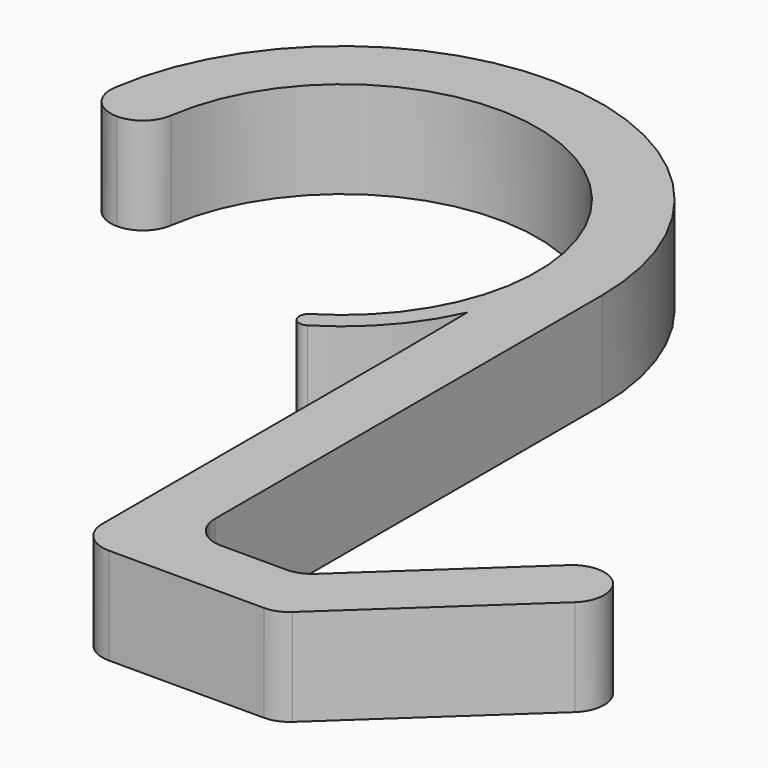
from build123d import *

# Parameters (mm, degrees)
F1_DEPTH    = 15
F2_T1_DEPTH = 15
F2_T3_DEPTH = 38.2179411812
F2_T5_DEPTH = 43.6185312436
F2_T7_DEPTH = 40
F2_T9_DEPTH = 24.832214185
F3_R        = 1.49999


# Not quite as in the source:
# - a fillet or chamfer that OpenCascade refuses, or shapes differently, is made with other operations: its cross-section is extruded or revolved along the edge and cut away or added
# - a fillet or chamfer is up to 0.001 mm smaller than in the source, because OpenCascade refuses the exact size


with BuildPart() as f1:
    # F0 (on Top) → F1 (new body)
    with BuildSketch(Plane.XY):
        with BuildLine():
            ThreePointArc((-30.25, 0), (15.4242466579, 26.0222042694), (14.5205861182, -26.5370510567))
            Line((14.5205861182, -26.5370510567), (15.9606442456, -29.1688247152))
            ThreePointArc((15.9606442456, -29.1688247152), (24.4038188383, -22.5835366164), (30.3161764706, -13.6562053369))
            Line((30.3161764706, -13.6562053369), (30.4329268293, -26.3419715398))
            Line((30.4329268293, -26.3419715398), (30.4329268293, -89.5091558098))
            Line((30.4329268293, -89.5091558098), (61.4327350343, -89.5091558098))
            Line((61.4327350343, -89.5091558098), (91.6112407267, -61.4279471198))
            Line((91.6112407267, -61.4279471198), (84.9590376288, -54.2789119314))
            Line((84.9590376288, -54.2789119314), (57.316922531, -80))
            Line((57.316922531, -80), (40.25, -80))
            Line((40.25, -80), (40.25, 0))
            ThreePointArc((40.25, 0), (0, 40.25), (-40.25, 0))
            Line((-40.25, 0), (-30.25, 0))
        make_face()
    extrude(amount=F1_DEPTH)

    # F2: fillet of radius 5 on 8 edges, made by hand

    # F2_s2 → F2_t1 (join)
    with BuildSketch(Plane.XY):
        with BuildLine():
            ThreePointArc((45.25, -80), (41.7144660941, -78.5355339059), (40.25, -75))
            Line((40.25, -75), (40.25, -80))
            Line((40.25, -80), (45.25, -80))
        make_face()
        with BuildLine():
            ThreePointArc((58.7565312825, -78.6604388503), (57.1804804794, -79.6530739437), (55.350479694, -80))
            Line((55.350479694, -80), (57.316922531, -80))
            Line((57.316922531, -80), (58.7565312825, -78.6604388503))
        make_face()
    extrude(amount=F2_T1_DEPTH)

    # F2_s4 → F2_t3 (cut)
    with BuildSketch(Plane.XY.offset(-11.6089705906)):
        with BuildLine():
            ThreePointArc((-29.9441430963, 4.2907801418), (-31.6183858983, 1.2220310158), (-34.8935882362, 0))
            Line((-34.8935882362, 0), (-30.25, 0))
            ThreePointArc((-30.25, 0), (-30.1734388881, 2.1508337146), (-29.9441430963, 4.2907801418))
        make_face()
    extrude(amount=F2_T3_DEPTH, mode=Mode.SUBTRACT)

    # F2_s6 → F2_t5 (cut)
    with BuildSketch(Plane.XY.offset(-14.3092656218)):
        with BuildLine():
            ThreePointArc((-34.8935882362, 0), (-38.6715572204, 1.724797662), (-39.8430333761, 5.7092198582))
            ThreePointArc((-39.8430333761, 5.7092198582), (-40.1481294296, 2.8618531244), (-40.25, 0))
            Line((-40.25, 0), (-34.8935882362, 0))
        make_face()
    extrude(amount=F2_T5_DEPTH, mode=Mode.SUBTRACT)

    # F2_s8 → F2_t7 (cut)
    with BuildSketch(Plane.XY.offset(-12.5)):
        with BuildLine():
            ThreePointArc((88.3650892173, -57.9393507817), (84.8845293249, -56.3486390617), (81.2985987785, -57.6849635199))
            Line((81.2985987785, -57.6849635199), (84.9590376288, -54.2789119314))
            Line((84.9590376288, -54.2789119314), (88.3650892173, -57.9393507817))
        make_face()
        with BuildLine():
            ThreePointArc((87.9508018764, -64.8339987083), (89.5415135964, -61.3534388159), (88.2051891382, -57.7675082695))
            Line((88.2051891382, -57.7675082695), (91.6112407267, -61.4279471198))
            Line((91.6112407267, -61.4279471198), (87.9508018764, -64.8339987083))
        make_face()
        with BuildLine():
            ThreePointArc((30.4329268293, -84.5091558098), (31.8973929233, -88.0446897157), (35.4329268293, -89.5091558098))
            Line((35.4329268293, -89.5091558098), (30.4329268293, -89.5091558098))
            Line((30.4329268293, -89.5091558098), (30.4329268293, -84.5091558098))
        make_face()
    extrude(amount=F2_T7_DEPTH, mode=Mode.SUBTRACT)

    # F2_s10 → F2_t9 (cut)
    with BuildSketch(Plane.XY.offset(-4.9161070925)):
        with BuildLine():
            ThreePointArc((59.4662921973, -89.5091558098), (61.2962929826, -89.1622297535), (62.8723437858, -88.1695946601))
            Line((62.8723437858, -88.1695946601), (61.4327350343, -89.5091558098))
            Line((61.4327350343, -89.5091558098), (59.4662921973, -89.5091558098))
        make_face()
    extrude(amount=F2_T9_DEPTH, mode=Mode.SUBTRACT)

    # F3 (radius 1.5 in the source; OpenCascade refuses exactly that, so slightly less here)
    f3_edges = [f1.edges().sort_by_distance(p)[0] for p in [
        (14.520586, -26.537051, 7.5),
        (15.960644, -29.168825, 7.5),
    ]]
    fillet(f3_edges, radius=F3_R)


solid = f1.part
